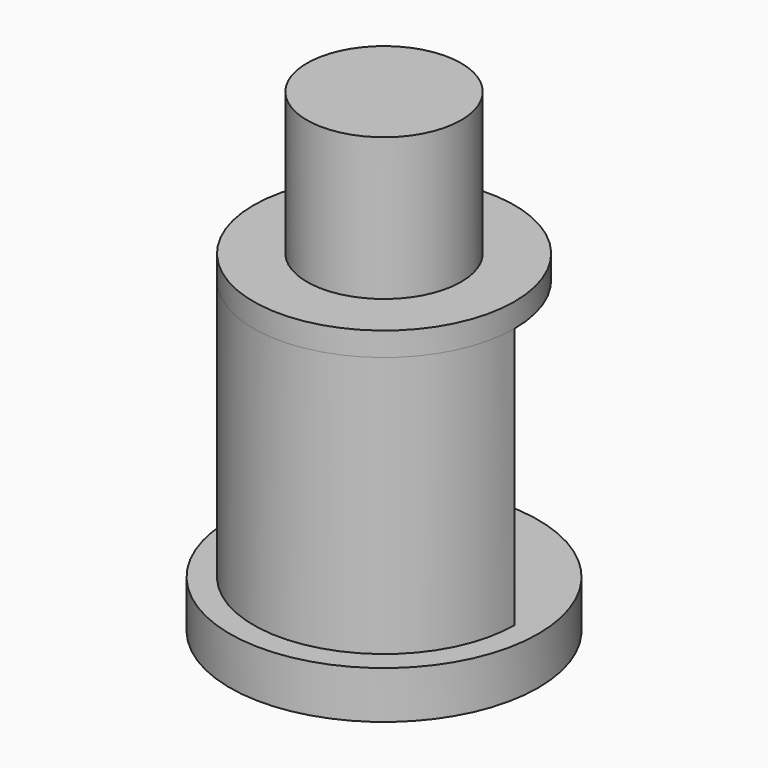
from build123d import *

# Parameters (mm, degrees)
F0_R      = 55
F0_R_2    = 45
F1_DEPTH  = 55
F3_DEPTH  = 130
F5_R      = 55
F6_DEPTH  = 10
F7_R      = 32.5
F8_DEPTH  = 70
F11_R     = 65
F12_DEPTH = 20


with BuildPart() as f1:
    # F0 (on Top) → F1 (new body, symmetric)
    with BuildSketch(Plane.XY):
        Circle(F0_R)
        Circle(F0_R_2, mode=Mode.SUBTRACT)
    extrude(amount=F1_DEPTH, both=True)

    # F2 (on face) → F3 (cut)
    with BuildSketch(Plane.XY.offset(55)):
        with BuildLine():
            ThreePointArc((-45, 0), (0, 45), (45, 0))
            Line((45, 0), (60, 0))
            ThreePointArc((60, 0), (0, 60), (-60, 0))
            Line((-60, 0), (-45, 0))
        make_face()
    extrude(amount=-F3_DEPTH, mode=Mode.SUBTRACT)

    # F11 (on offset) → F12 (join)
    with BuildSketch(Plane(origin=(0, 0, -55), x_dir=(1, 0, 0), z_dir=(0, 0, -1))):
        Circle(F11_R)
    extrude(amount=F12_DEPTH)


with BuildPart() as f6:
    # F5 (on offset) → F6 (new body)
    with BuildSketch(Plane.XY.offset(55)):
        Circle(F5_R)
    extrude(amount=F6_DEPTH)


with BuildPart() as f8:
    # F7 (on offset) → F8 (new body)
    with BuildSketch(Plane.XY.offset(55)):
        Circle(F7_R)
    extrude(amount=F8_DEPTH)


solid = Compound([f1.part, f6.part, f8.part])
